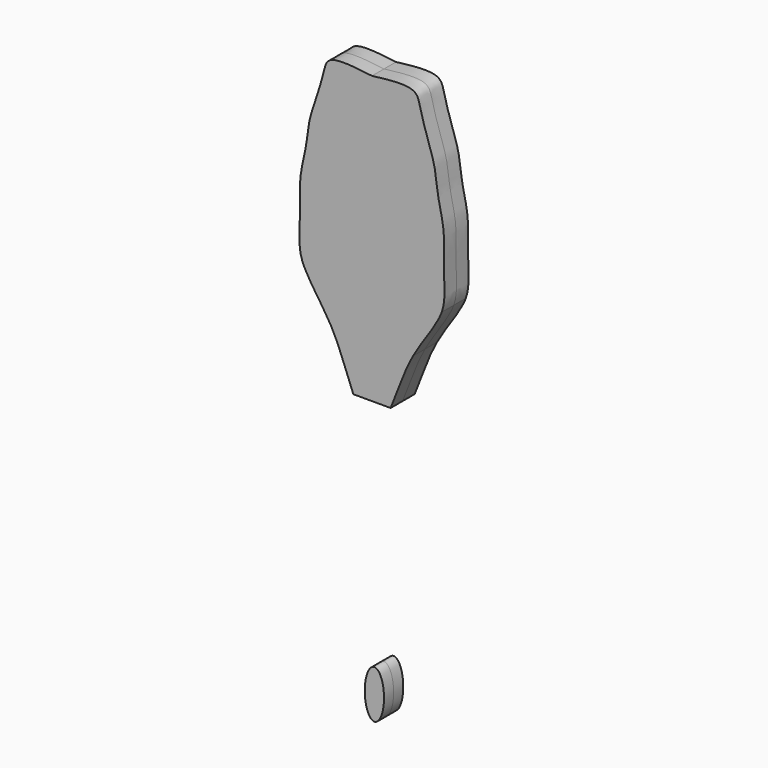
from build123d import *

# Parameters (mm, degrees)
F4_DEPTH = 5
F5_DEPTH = 6.25


# Not quite as in the source:
# - a feature of the source that left no trace in its solid (it failed there, or was rolled back) is left out
# - the program builds the solid bodies; features that only make, move or delete a surface that nothing else refers to are left out


with BuildPart() as f4:
    # F3 (on Front) → F4 (new body, symmetric)
    with BuildSketch(Plane.XZ):
        with BuildLine():
            add(Edge.make_bspline(
                [(0, -139.7883538913), (6.9282032303, -139.7883538913), (3.4641016151, -124.7883538913), (0, -109.7883538913), (-3.4641016151, -124.7883538913), (-6.9282032303, -139.7883538913), (0, -139.7883538913)],
                knots=[0, 0, 0, 2.0943951024, 2.0943951024, 4.1887902048, 4.1887902048, 6.2831853072, 6.2831853072, 6.2831853072], degree=2, weights=[1, 0.5, 1, 0.5, 1, 0.5, 1]))
        make_face()
    extrude(amount=F4_DEPTH, both=True)


with BuildPart() as f5:
    # F0 (on Front) → F5 (new body, symmetric)
    with BuildSketch(Plane.XZ):
        with BuildLine():
            add(Edge.make_bspline(
                [(0, 0), (-6.1817182185, 1.5497331273), (-16.6267945213, 4.1682738294), (-21.2329716017, 7.7883473251), (-23, 10)],
                knots=[0, 0, 0, 0, 0.3980714095, 0.6726101222, 0.6726101222, 0.6726101222, 0.6726101222], degree=3))
            Line((0, 0), (0, 10))
            Line((0, 10), (-23, 10))
        make_face()
        with BuildLine():
            Line((-17, 0), (0, 0))
            add(Edge.make_bspline(
                [(0, 0), (-6.1817182185, 1.5497331273), (-16.6267945213, 4.1682738294), (-21.2329716017, 7.7883473251), (-23, 10)],
                knots=[0, 0, 0, 0, 0.3980714095, 0.6726101222, 0.6726101222, 0.6726101222, 0.6726101222], degree=3))
            add(Edge.make_bspline(
                [(-23, 10), (-25.1071972174, 12.6374156561), (-27.0535986087, 16.318707828), (-29, 20)],
                knots=[0.6726101222, 0.6726101222, 0.6726101222, 0.6726101222, 1, 1, 1, 1], degree=3))
            add(Edge.make_bspline(
                [(-17, 0), (-21.2383851929, 7.571398185), (-26.9372982981, 14.2138719481), (-29, 20)],
                knots=[0, 0, 0, 0, 0.1419768486, 0.1419768486, 0.1419768486, 0.1419768486], degree=3))
        make_face()
        with BuildLine():
            Line((17, 0), (0, 0))
            Line((0, 0), (-17, 0))
            add(Edge.make_bspline(
                [(-17, 0), (-16.0155350041, -1.7586359295), (-15.134084666, -3.5675646177), (-14.3165010119, -5.4076736428)],
                knots=[0, 0, 0, 0, 6.0463001038, 6.0463001038, 6.0463001038, 6.0463001038], degree=3))
            add(Edge.make_bspline(
                [(-7.75, -22), (-8.6932001461, -17.4038997455), (-11.3156170337, -11.5477802243), (-14.3165010119, -5.4076736428)],
                knots=[0.8975094294, 0.8975094294, 0.8975094294, 0.8975094294, 0.9769003565, 0.9769003565, 0.9769003565, 0.9769003565], degree=3))
            Line((-7.75, -22), (0, -22))
            Line((0, -22), (7.75, -22))
            add(Edge.make_bspline(
                [(17, 0), (13.1141925793, -6.9415576719), (10.8333333333, -14.6666666667), (7.75, -22)],
                knots=[0, 0, 0, 0, 23.8655085846, 23.8655085846, 23.8655085846, 23.8655085846], degree=3))
        make_face()
        with BuildLine():
            Line((0, 10), (0, 0))
            add(Edge.make_bspline(
                [(0, 0), (6.1817182185, 1.5497331273), (16.6267945213, 4.1682738294), (21.2329716017, 7.7883473251), (23, 10)],
                knots=[0, 0, 0, 0, 0.3980714095, 0.6726101222, 0.6726101222, 0.6726101222, 0.6726101222], degree=3))
            Line((23, 10), (0, 10))
        make_face()
        with BuildLine():
            add(Edge.make_bspline(
                [(0, 0), (6.1817182185, 1.5497331273), (16.6267945213, 4.1682738294), (21.2329716017, 7.7883473251), (23, 10)],
                knots=[0, 0, 0, 0, 0.3980714095, 0.6726101222, 0.6726101222, 0.6726101222, 0.6726101222], degree=3))
            Line((0, 0), (17, 0))
            add(Edge.make_bspline(
                [(17, 0), (21.2383851929, 7.571398185), (26.9372982981, 14.2138719481), (29, 20)],
                knots=[0, 0, 0, 0, 0.1419768486, 0.1419768486, 0.1419768486, 0.1419768486], degree=3))
            add(Edge.make_bspline(
                [(23, 10), (25.1071972174, 12.6374156561), (27.0535986087, 16.318707828), (29, 20)],
                knots=[0.6726101222, 0.6726101222, 0.6726101222, 0.6726101222, 1, 1, 1, 1], degree=3))
        make_face()
        with BuildLine():
            Line((-23, 10), (0, 10))
            Line((0, 10), (0, 20))
            Line((0, 20), (0, 22))
            Line((0, 22), (0, 32))
            Line((0, 32), (0, 42))
            Line((0, 42), (0, 52))
            Line((0, 52), (0, 62))
            Line((0, 62), (0, 72))
            Line((0, 72), (0, 82))
            Line((0, 82), (0, 92))
            Line((0, 92), (0, 97))
            add(Edge.make_bspline(
                [(-29, 20), (-30.4410186861, 24.0422319112), (-29.7845042484, 31.1738104083), (-30.06719671, 41.9849282884), (-29.9378480605, 52.0397662603), (-27.155594339, 61.9495686988), (-26.4447656669, 72.1472686821), (-22.9889862534, 81.8172313094), (-19.8856790399, 91.6678357607), (-18.6439473926, 99.252081713), (-7.2680581597, 97.8779416175), (0, 97)],
                knots=[0.1419768486, 0.1419768486, 0.1419768486, 0.1419768486, 0.2411629265, 0.3371469979, 0.4301696896, 0.5240503513, 0.6175335655, 0.7125228096, 0.8075120536, 0.8770193366, 1, 1, 1, 1], degree=3))
            add(Edge.make_bspline(
                [(-23, 10), (-25.1071972174, 12.6374156561), (-27.0535986087, 16.318707828), (-29, 20)],
                knots=[0.6726101222, 0.6726101222, 0.6726101222, 0.6726101222, 1, 1, 1, 1], degree=3))
        make_face()
        with BuildLine():
            Line((0, 20), (0, 10))
            Line((0, 10), (23, 10))
            add(Edge.make_bspline(
                [(23, 10), (25.1071972174, 12.6374156561), (27.0535986087, 16.318707828), (29, 20)],
                knots=[0.6726101222, 0.6726101222, 0.6726101222, 0.6726101222, 1, 1, 1, 1], degree=3))
            add(Edge.make_bspline(
                [(29, 20), (30.4410186861, 24.0422319112), (29.7845042484, 31.1738104083), (30.06719671, 41.9849282884), (29.9378480605, 52.0397662603), (27.155594339, 61.9495686988), (26.4447656669, 72.1472686821), (22.9889862534, 81.8172313094), (19.8856790399, 91.6678357607), (18.6439473926, 99.252081713), (7.2680581597, 97.8779416175), (0, 97)],
                knots=[0.1419768486, 0.1419768486, 0.1419768486, 0.1419768486, 0.2411629265, 0.3371469979, 0.4301696896, 0.5240503513, 0.6175335655, 0.7125228096, 0.8075120536, 0.8770193366, 1, 1, 1, 1], degree=3))
            Line((0, 97), (0, 92))
            Line((0, 92), (0, 82))
            Line((0, 82), (0, 72))
            Line((0, 72), (0, 62))
            Line((0, 62), (0, 52))
            Line((0, 52), (0, 42))
            Line((0, 42), (0, 32))
            Line((0, 32), (0, 22))
            Line((0, 22), (0, 20))
        make_face()
        with BuildLine():
            add(Edge.make_bspline(
                [(-7.75, -22), (-8.6932001461, -17.4038997455), (-11.3156170337, -11.5477802243), (-14.3165010119, -5.4076736428)],
                knots=[0.8975094294, 0.8975094294, 0.8975094294, 0.8975094294, 0.9769003565, 0.9769003565, 0.9769003565, 0.9769003565], degree=3))
            add(Edge.make_bspline(
                [(-14.3165010119, -5.4076736428), (-11.906978935, -10.8307068669), (-10.0521742565, -16.524558525), (-7.75, -22)],
                knots=[6.0463001038, 6.0463001038, 6.0463001038, 6.0463001038, 23.8655085846, 23.8655085846, 23.8655085846, 23.8655085846], degree=3))
        make_face()
    extrude(amount=F5_DEPTH, both=True)


solid = Compound([f4.part, f5.part])
